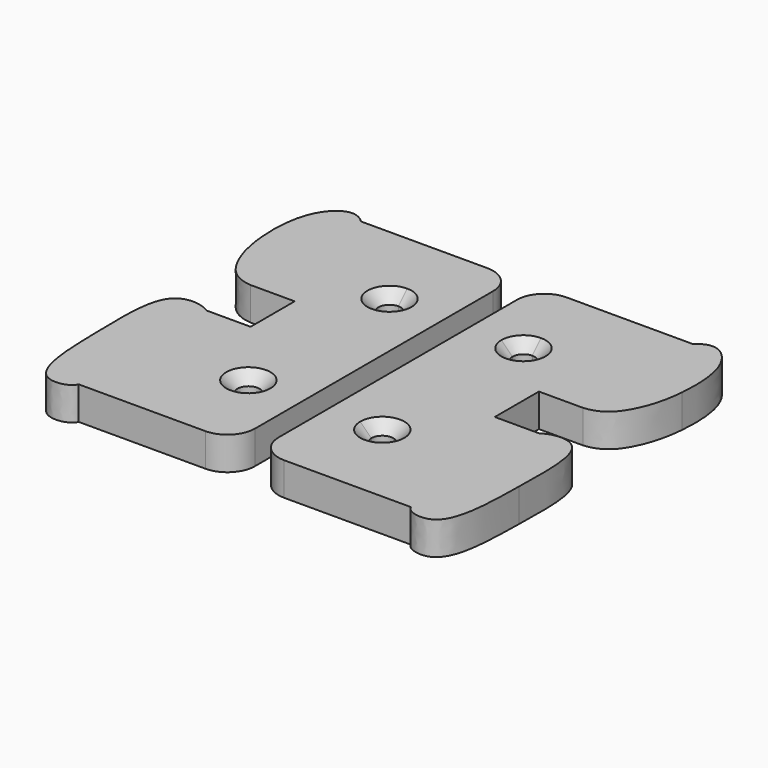
from build123d import *

# Parameters (mm, degrees)
F1_DEPTH = 7.62
F2_R     = 6.35
F3_SIZE  = 2.54


with BuildPart() as f1:
    # F0 (on Top) → F1 (new body)
    with BuildSketch(Plane.XY):
        Polygon((0, 18.415), (0, 0), (12.7, 0), (25.4, 0), (25.4, 81.28), (12.7, 81.28), (0, 81.28), (0, 65.405), (0, 49.53), (0, 36.83), align=None)
        with BuildLine():
            ThreePointArc((15.24, 20.32), (14.4960512242, 18.5239487758), (12.7, 17.78))
            ThreePointArc((12.7, 17.78), (10.9039487758, 22.1160512242), (15.24, 20.32))
        make_face(mode=Mode.SUBTRACT)
        with BuildLine():
            ThreePointArc((15.24, 60.96), (10.9039487758, 59.1639487758), (12.7, 63.5))
            ThreePointArc((12.7, 63.5), (14.4960512242, 62.7560512242), (15.24, 60.96))
        make_face(mode=Mode.SUBTRACT)
        with BuildLine():
            Line((-10.16, 49.53), (0, 49.53))
            Line((0, 49.53), (0, 65.405))
            Line((0, 65.405), (-20.32, 65.405))
            add(Edge.make_bspline(
                [(-10.16, 49.53), (-14.331649676, 49.8729012967), (-18.3920992899, 55.1877378663), (-19.9701763147, 61.4448046081), (-20.32, 65.405)],
                knots=[0, 0, 0, 0, 0.2379462848, 0.4877519456, 0.4877519456, 0.4877519456, 0.4877519456], degree=3))
        make_face()
        with BuildLine():
            Line((-20.32, 65.405), (0, 65.405))
            Line((0, 65.405), (0, 81.28))
            Line((0, 81.28), (-10.16, 81.28))
            add(Edge.make_bspline(
                [(-20.32, 65.405), (-20.7295661244, 70.0415124684), (-20.3463914547, 79.9762511033), (-13.1395673379, 84.3035876751), (-10.16, 81.28)],
                knots=[0.4877519456, 0.4877519456, 0.4877519456, 0.4877519456, 0.780219096, 1, 1, 1, 1], degree=3))
        make_face()
        with BuildLine():
            Line((-20.32, 18.415), (0, 18.415))
            Line((0, 18.415), (0, 36.83))
            Line((0, 36.83), (-10.16, 36.83))
            add(Edge.make_bspline(
                [(-20.32, 18.415), (-20.4827266675, 26.5430610833), (-20.9380249073, 38.955794752), (-12.4576338451, 38.3399460251), (-10.16, 36.83)],
                knots=[0.4971306325, 0.4971306325, 0.4971306325, 0.4971306325, 0.8044152788, 1, 1, 1, 1], degree=3))
        make_face()
        with BuildLine():
            Line((-10.16, 0), (0, 0))
            Line((0, 0), (0, 18.415))
            Line((0, 18.415), (-20.32, 18.415))
            add(Edge.make_bspline(
                [(-10.16, 0), (-10.7667939737, -1.6637903173), (-20.0818121137, -4.1002458839), (-20.1507904755, 9.9631256242), (-20.32, 18.415)],
                knots=[0, 0, 0, 0, 0.1776040933, 0.4971306325, 0.4971306325, 0.4971306325, 0.4971306325], degree=3))
        make_face()
    extrude(amount=F1_DEPTH)

    # F2
    f2_edges = [f1.edges().sort_by_distance(p)[0] for p in [
        (25.4, 0, 3.81),
        (25.4, 81.28, 3.81),
    ]]
    fillet(f2_edges, radius=F2_R)

    # F3
    f3_edges = [f1.edges().sort_by_distance(p)[0] for p in [
        (10.16, 60.96, 7.62),
        (12.7, 22.86, 7.62),
    ]]
    chamfer(f3_edges, length=F3_SIZE)


with BuildPart() as f6_1:
    # F6: instance of F1
    add(f1.part.mirror(Plane(origin=(28.1277354807, 41.8248549104, 12.7), x_dir=(0, 1, 0), z_dir=(1, 0, 0))))


solid = Compound([f1.part, f6_1.part])
